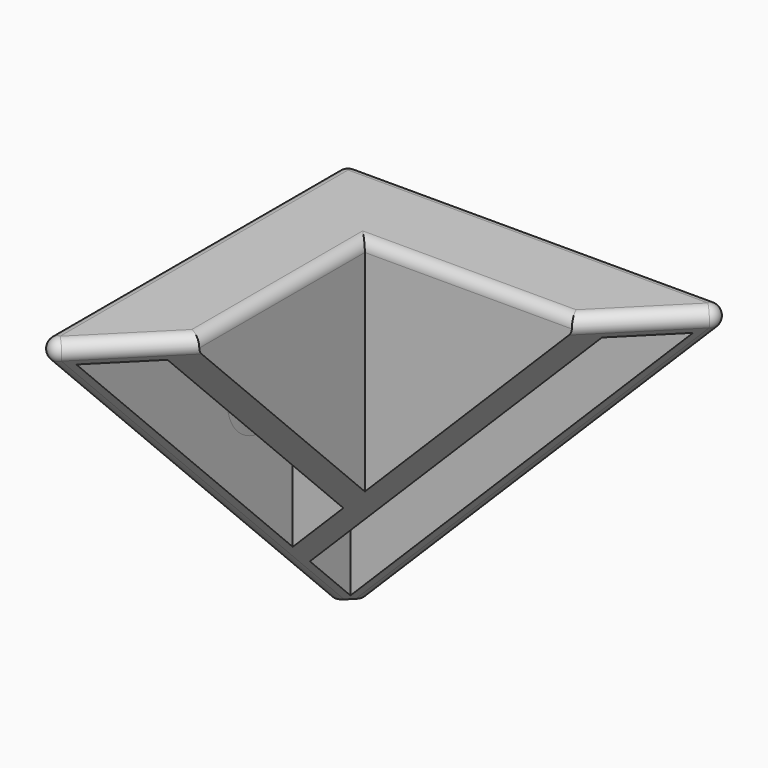
from build123d import *

# Parameters (mm, degrees)
F1_DEPTH  = 28.575
F3_R      = 38.1
F4_DEPTH  = 32.9965678842
F6_W      = 26.9748
F6_H      = 3.5145800794
F6_W_2    = 3.5145800794
F6_H_2    = 21.971
F7_DEPTH  = 26.9758
F8_R      = 0.762
F15_W     = 1.8396307345
F15_H     = 1.8396307345
F16_DEPTH = 26.4941772846


# Not quite as in the source:
# - a fillet or chamfer that OpenCascade refuses, or shapes differently, is made with other operations: its cross-section is extruded or revolved along the edge and cut away or added
# - a pattern or mirror of a feature is missing from the dataset's text; its kind, count and spacing are read off the source's solid


with BuildPart() as f1:
    # F0 (on Top) → F1 (new body)
    with BuildSketch(Plane.XY):
        Polygon((0, -21.971), (0, 0), (21.971, 0), (21.971, 6.604), (-6.604, 6.604), (-6.604, -21.971), align=None)
    extrude(amount=-F1_DEPTH)

    # F3 (on 3pt) → F4 (cut, through all)
    with BuildSketch(Plane(origin=(5.1223333333, -5.1223333333, -5.1223333333), x_dir=(0.8164965809, 0.4082482905, 0.4082482905), z_dir=(0.5773502692, -0.5773502692, -0.5773502692))):
        Circle(F3_R)
    extrude(amount=F4_DEPTH, mode=Mode.SUBTRACT)

    # F6 (on offset) → F7 (cut, through all)
    with BuildSketch(Plane.XY.offset(-1.6002)):
        with Locations((8.4836, 3.2465099603)):
            Rectangle(F6_W, F6_H)
        with Locations((-3.2465099603, -10.9855)):
            Rectangle(F6_W_2, F6_H_2)
    extrude(amount=-F7_DEPTH, mode=Mode.SUBTRACT)

    # F8
    f8_edges = [f1.edges().sort_by_distance(p)[0] for p in [
        (7.6835, 6.604, 0),
        (18.669, 3.302, 0),
        (7.6835, 0, 0),
        (0, -7.6835, 0),
        (-3.302, -18.669, 0),
        (-6.604, -7.6835, 0),
        (-6.604, 6.604, -14.2875),
        (7.6835, 6.604, -14.2875),
        (-6.604, -7.6835, -14.2875),
    ]]
    fillet(f8_edges, radius=F8_R)

    # F10 (on offset) → F11 (revolve)
    with BuildSketch(Plane.YZ.offset(2.6162)):
        with BuildLine():
            ThreePointArc((4.2418, -9.2202), (4.4469151823, -9.9607308906), (5.0038, -10.4902))
            Line((5.0038, -10.4902), (5.0038, -9.2202))
            Line((5.0038, -9.2202), (4.2418, -9.2202))
        make_face()
    f11 = revolve(axis=Axis((2.6162, 4.6228, -9.2202), (0, -1, 0)))

    # F11_copies: F11 across plane
    add(f11.mirror(Plane(origin=(0, 0, 0), x_dir=(0.7071067796, -0.7071067828, 0), z_dir=(-0.7071067828, -0.7071067796, 0))))

    # F14: fillet of radius 5.08 on 3 edges, made by hand

    # F14_s1 → F14_t2 (revolve)
    with BuildSketch(Plane.YZ.offset(2.6162)):
        with BuildLine():
            ThreePointArc((5.0038, -12.278765023), (4.853123865, -11.0506908258), (4.4100337662, -9.8954676025))
            ThreePointArc((4.4100337662, -9.8954676025), (4.662543942, -10.2371346569), (5.0038, -10.4902))
            Line((5.0038, -10.4902), (5.0038, -12.278765023))
        make_face()
    revolve(axis=Axis((2.6162, 5.0038, -9.2202), (0, -1, 0)))

    # F14_s3 → F14_t4 (revolve)
    with BuildSketch(Plane.XZ.offset(2.6161999777)):
        with BuildLine():
            ThreePointArc((-5.0038, -12.2787650011), (-4.8531238674, -11.0506908133), (-4.4100337753, -9.8954675976))
            ThreePointArc((-4.4100337753, -9.8954675976), (-4.6625439517, -10.237134655), (-5.0038000116, -10.4902))
            Line((-5.0038000116, -10.4902), (-5.0038, -12.2787650011))
        make_face()
    revolve(axis=Axis((-5.0038000116, -2.6161999777, -9.2202), (-1, 4.4e-09, 0)))

    # F15 (on face) → F16 (cut, through all)
    with BuildSketch(Plane(origin=(-6.604, 0, 0), x_dir=(0, -1, 0), z_dir=(-1, 0, 0))):
        with Locations((-5.6841846327, -26.6509926519)):
            Rectangle(F15_W, F15_H)
    extrude(amount=-F16_DEPTH, mode=Mode.SUBTRACT)


solid = f1.part
